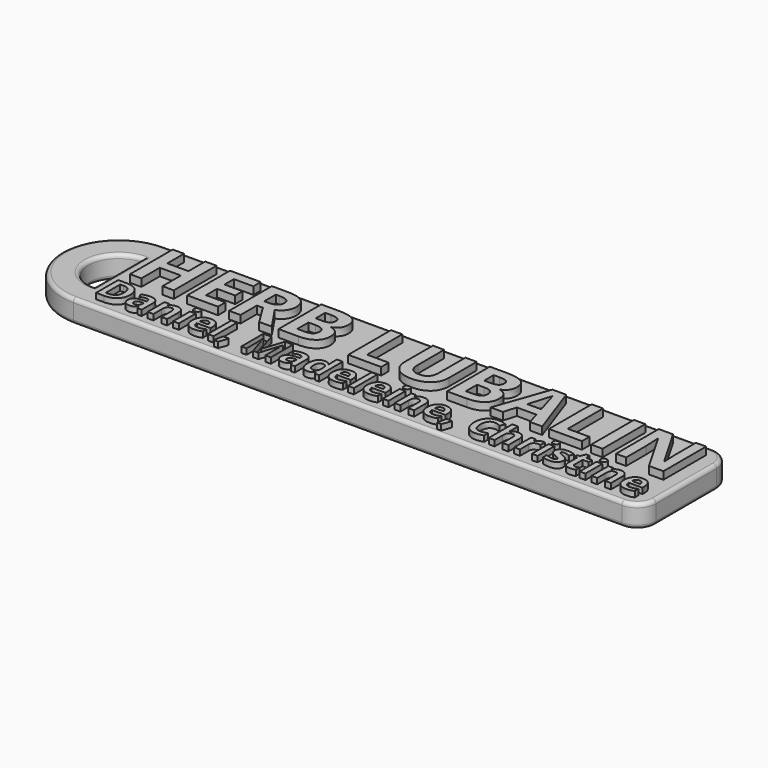
from build123d import *

# Parameters (mm, degrees)
F1_DEPTH     = 3
F2_TEXT_SIZE = 9.8848059721
F3_DEPTH     = 1
F4_TEXT_SIZE = 5.113068951
F5_DEPTH     = 0.75
F6_R         = 2.5
F7_R         = 0.5


# Not quite as in the source:
# - Text() gives the source's letters only with a copy of the font that has no kerning and outlines rounded to 1/6400 em; it was checked with that copy


with BuildPart() as f1:
    # F0 (on Top) → F1 (new body)
    with BuildSketch(Plane.XY):
        Polygon((-37.5, -7.5), (37.5, -7.5), (37.5, 7.5), (-37.5, 7.5), (-37.5, 4), (-37.5, -4), align=None)
        with BuildLine():
            ThreePointArc((-37.5, 7.5), (-45, 0), (-37.5, -7.5))
            Line((-37.5, -7.5), (-37.5, -4))
            ThreePointArc((-37.5, -4), (-41.5, 0), (-37.5, 4))
            Line((-37.5, 4), (-37.5, 7.5))
        make_face()
    extrude(amount=F1_DEPTH)

    # F2 (on face) → F3 (join)
    with BuildSketch(Plane.XY.offset(3)):
        with Locations((-36, -1.1170602999)):
            Text('HERB LUBALIN', F2_TEXT_SIZE, font='Open Sans', font_style=FontStyle.BOLD, text_align=(TextAlign.LEFT, TextAlign.BOTTOM))
    extrude(amount=F3_DEPTH)

    # F4 (on face) → F5 (join)
    with BuildSketch(Plane.XY.offset(3)):
        with Locations((-36, -6.1814096447)):
            Text('Daniel, Madeleine, Christine', F4_TEXT_SIZE, font='Open Sans', font_style=FontStyle.BOLD, text_align=(TextAlign.LEFT, TextAlign.BOTTOM))
    extrude(amount=F5_DEPTH)

    # F6
    f6_edges = [f1.edges().sort_by_distance(p)[0] for p in [
        (37.5, 7.5, 1.5),
        (37.5, -7.5, 1.5),
    ]]
    fillet(f6_edges, radius=F6_R)

    # F7
    f7_edges = [f1.edges().sort_by_distance(p)[0] for p in [
        (-45, 0, 3),
        (-41.5, 0, 3),
        (-37.5, 0, 3),
        (-45, 0, 0),
        (-41.5, 0, 0),
        (-37.5, 0, 0),
    ]]
    fillet(f7_edges, radius=F7_R)


solid = f1.part
